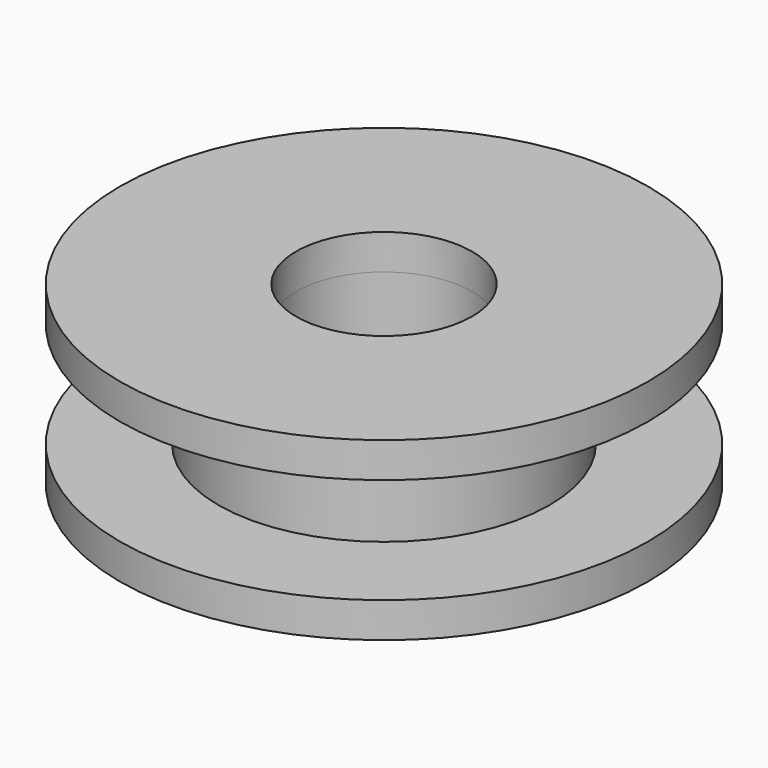
from build123d import *

# Parameters (mm, degrees)
F0_R     = 7.5
F0_R_2   = 3.5
F0_R_3   = 2.5
F1_DEPTH = 1
F2_R     = 3.5
F2_R_2   = 2.5
F3_DEPTH = 3
F4_R     = 4.7
F4_R_2   = 3.7
F5_DEPTH = 3
F4_R_3   = 7.5
F4_R_4   = 3.5
F4_R_5   = 2.5
F6_DEPTH = 1


with BuildPart() as f1:
    # F0 (on Top) → F1 (new body)
    with BuildSketch(Plane.XY):
        Circle(F0_R)
        Circle(F0_R_2, mode=Mode.SUBTRACT)
        Circle(F0_R_2)
        Circle(F0_R_3, mode=Mode.SUBTRACT)
    extrude(amount=F1_DEPTH)

    # F2 (on face) → F3 (join)
    with BuildSketch(Plane.XY.offset(1)):
        Circle(F2_R)
        Circle(F2_R_2, mode=Mode.SUBTRACT)
    extrude(amount=F3_DEPTH)


with BuildPart() as f5:
    # F4 (on face) → F5 (new body, through all)
    with BuildSketch(Plane.XY.offset(4)):
        Circle(F4_R)
        Circle(F4_R_2, mode=Mode.SUBTRACT)
    extrude(amount=-F5_DEPTH)

    # F4 (on face) → F6 (join)
    with BuildSketch(Plane.XY.offset(4)):
        Circle(F4_R_3)
        Circle(F4_R, mode=Mode.SUBTRACT)
        Circle(F4_R)
        Circle(F4_R_2, mode=Mode.SUBTRACT)
        Circle(F4_R_2)
        Circle(F4_R_4, mode=Mode.SUBTRACT)
        Circle(F4_R_4)
        Circle(F4_R_5, mode=Mode.SUBTRACT)
    extrude(amount=F6_DEPTH)


solid = Compound([f1.part, f5.part])
